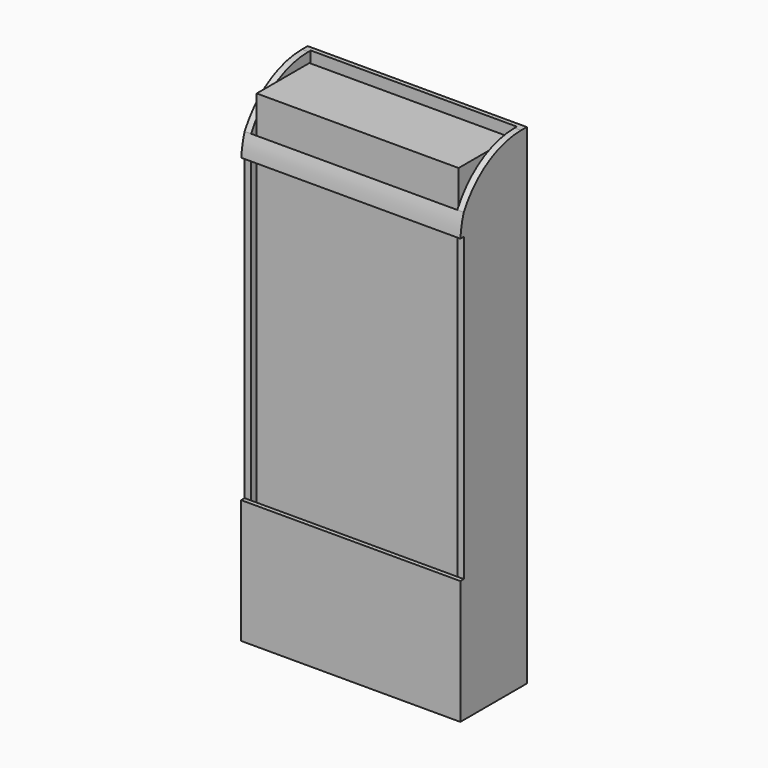
from build123d import *

# Parameters (mm, degrees)
F0_W         = 46.9
F0_H         = 109.8
F1_DEPTH     = 15.3
F3_W         = 50.9
F3_H         = 113.8
F4_DEPTH     = 1
F8_W         = 50.9
F8_H         = 113.8
F9_DEPTH     = 1
F6_W         = 50.9
F6_H         = 113.8
F6_W_2       = 47.9
F6_H_2       = 110.8
F10_DEPTH    = 17.3
F12_W        = 50.9
F12_H        = 85
F13_DEPTH    = 25
F14_W        = 47.9
F14_H        = 10.7243023813
F15_DEPTH    = 17.3
F16_W        = 50.9
F16_H        = 5
F17_DEPTH    = 1
F18_T1_DEPTH = 84.6590818447
F18_T3_DEPTH = 84.6590818447
F18_T5_DEPTH = 81.1744659627


# Not quite as in the source:
# - a fillet or chamfer that OpenCascade refuses, or shapes differently, is made with other operations: its cross-section is extruded or revolved along the edge and cut away or added


with BuildPart() as f1:
    # F0 (on Front) → F1 (new body)
    with BuildSketch(Plane.XZ):
        Rectangle(F0_W, F0_H)
    extrude(amount=F1_DEPTH)


with BuildPart() as f4:
    # F3 (on offset) → F4 (new body)
    with BuildSketch(Plane.XZ.offset(-1)):
        Rectangle(F3_W, F3_H)
    extrude(amount=-F4_DEPTH)



with BuildPart() as f9:
    # F8 (on offset) → F9 (new body)
    with BuildSketch(Plane.XZ.offset(16.3)):
        Rectangle(F8_W, F8_H)
    extrude(amount=F9_DEPTH)


with BuildPart() as f4_1:
    add(f4.part)

    add(f9.part)  # F10 merges F9
    # F6 (on offset) → F10 (join, through all)
    with BuildSketch(Plane.XZ.offset(-1)):
        Rectangle(F6_W, F6_H)
        Rectangle(F6_W_2, F6_H_2, mode=Mode.SUBTRACT)
    extrude(amount=F10_DEPTH)

    # F12 (on offset) → F13 (cut, through all)
    with BuildSketch(Plane.XZ.offset(41.3)):
        with Locations((0, 14.4)):
            Rectangle(F12_W, F12_H)
    extrude(amount=-F13_DEPTH, mode=Mode.SUBTRACT)

    # F14 (on offset) → F15 (cut, through all)
    with BuildSketch(Plane.XZ.offset(16.3)):
        with Locations((0, 52.6752341539)):
            Rectangle(F14_W, F14_H)
    extrude(amount=-F15_DEPTH, mode=Mode.SUBTRACT)

    # F16 (on offset) → F17 (join)
    with BuildSketch(Plane.XZ.offset(16.3)):
        with Locations((0, 44.4)):
            Rectangle(F16_W, F16_H)
    extrude(amount=F17_DEPTH)

    # F18: fillet of radius 18.8308657865 on 3 edges, made by hand

    # F18_s2 → F18_t1 (cut)
    with BuildSketch(Plane.YZ.offset(-17.6295409224)):
        with BuildLine():
            ThreePointArc((0.3318163689, 56.9), (-9.3714989888, 54.2075101335), (-16.3, 46.9))
            Line((-16.3, 46.9), (-16.3, 56.9))
            Line((-16.3, 56.9), (0.3318163689, 56.9))
        make_face()
    extrude(amount=F18_T1_DEPTH, mode=Mode.SUBTRACT)

    # F18_s4 → F18_t3 (cut)
    with BuildSketch(Plane.YZ.offset(-67.0295409224)):
        with BuildLine():
            ThreePointArc((0.3318163689, 56.9), (-9.3714989888, 54.2075101335), (-16.3, 46.9))
            Line((-16.3, 46.9), (-16.3, 56.9))
            Line((-16.3, 56.9), (0.3318163689, 56.9))
        make_face()
    extrude(amount=F18_T3_DEPTH, mode=Mode.SUBTRACT)

    # F18_s6 → F18_t5 (cut)
    with BuildSketch(Plane.YZ.offset(-40.5872329814)):
        with BuildLine():
            ThreePointArc((-16.3, 46.9), (-17.0483180862, 43.913564546), (-17.3, 40.8451068075))
            Line((-17.3, 40.8451068075), (-17.3, 46.9))
            Line((-17.3, 46.9), (-16.3, 46.9))
        make_face()
    extrude(amount=F18_T5_DEPTH, mode=Mode.SUBTRACT)


solid = Compound([f1.part, f4_1.part])
